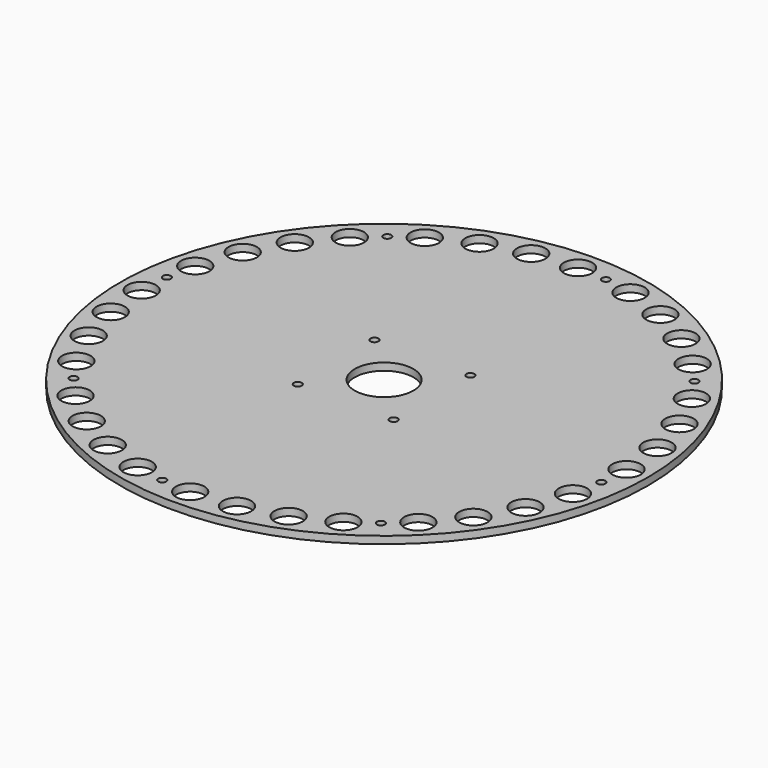
from build123d import *

# Parameters (mm, degrees)
F0_R            = 114.3
F0_R_2          = 1.7272
F0_R_3          = 12.7
F1_DEPTH        = 3.175
F2_R            = 6.1483621
F2_R_2          = 1.7272
F3_DEPTH        = 3.175
F3_COPIES_COUNT = 8


# Not quite as in the source:
# - a pattern or mirror of a feature is missing from the dataset's text; its kind, count and spacing are read off the source's solid


with BuildPart() as f1:
    # F0 (on Top) → F1 (new body)
    with BuildSketch(Plane.XY):
        Circle(F0_R)
        with Locations((-20.76684228, -20.76684228)):
            Circle(F0_R_2, mode=Mode.SUBTRACT)
        with Locations((20.76684228, -20.76684228)):
            Circle(F0_R_2, mode=Mode.SUBTRACT)
        with Locations((-20.76684228, 20.76684228)):
            Circle(F0_R_2, mode=Mode.SUBTRACT)
        Circle(F0_R_3, mode=Mode.SUBTRACT)
        with Locations((20.76684228, 20.76684228)):
            Circle(F0_R_2, mode=Mode.SUBTRACT)
    extrude(amount=F1_DEPTH)

    # F2 (on face) → F3 (cut, through all)
    with BuildSketch(Plane.XY.offset(3.175)):
        with Locations((-104.9766379, 0)):
            Circle(F2_R)
        with Locations((-103.2599191691, -18.9072366561)):
            Circle(F2_R)
        with Locations((-98.1659111494, -37.1960803446)):
            Circle(F2_R)
        with Locations((-89.8612219386, -54.2683636799)):
            Circle(F2_R)
        with Locations((-104.2084193553, 12.676744072)):
            Circle(F2_R_2)
    f3 = extrude(amount=-F3_DEPTH, mode=Mode.SUBTRACT)

    # F3_copies: F3 ×8 about axis
    f3_copies_axis = Axis((0, 0, 0), (0, 0, 1))
    for i in range(1, F3_COPIES_COUNT):
        add(f3.rotate(f3_copies_axis, i * 360 / F3_COPIES_COUNT), mode=Mode.SUBTRACT)


solid = f1.part
